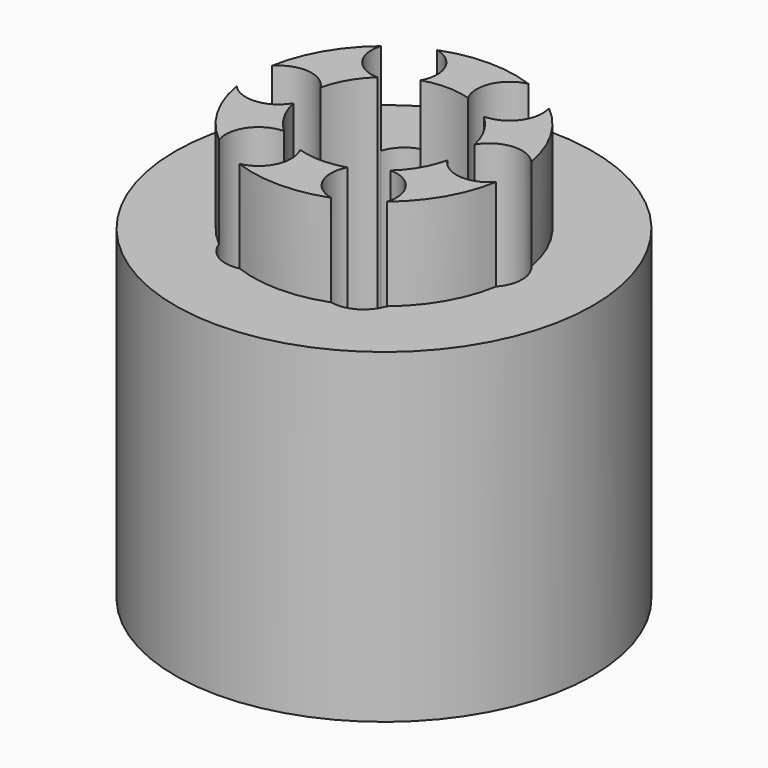
from build123d import *

# Parameters (mm, degrees)
F1_DEPTH = 3.175
F0_R     = 1.5875
F2_DEPTH = 2.475


# Not quite as in the source:
# - a length typed as a fraction of an inch, garbled in the dataset ("3 / 203.2 mm" for 3/8 in), is restored


with BuildPart() as f1:
    # F0 (on Top) → F1 (new body)
    with BuildSketch(Plane.XY):
        with BuildLine():
            ThreePointArc((-0.5859375, 0.1291404123), (-0.5196152423, 0.3), (-0.4048076277, 0.4428665539))
            ThreePointArc((-0.4048076277, 0.4428665539), (-0.6037234698, 0.5479177769), (-0.6376941264, 0.7702896865))
            ThreePointArc((-0.6376941264, 0.7702896865), (-0.8660254038, 0.5), (-0.9859375, 0.16711447))
            ThreePointArc((-0.9859375, 0.16711447), (-0.7763724489, 0.2488809732), (-0.5859375, 0.1291404123))
        make_face()
    extrude(amount=F1_DEPTH)



with BuildPart() as f1b:
    # F0 (on Top) → F1, piece 2 (new body)
    with BuildSketch(Plane.XY):
        with BuildLine():
            ThreePointArc((-0.1811298723, 0.5720069662), (0, 0.6), (0.1811298723, 0.5720069662))
            ThreePointArc((0.1811298723, 0.5720069662), (0.1726489791, 0.7967987502), (0.3482433736, 0.9374041566))
            ThreePointArc((0.3482433736, 0.9374041566), (0, 1), (-0.3482433736, 0.9374041566))
            ThreePointArc((-0.3482433736, 0.9374041566), (-0.2057847115, 0.8502383071), (-0.15, 0.692820323))
            ThreePointArc((-0.15, 0.692820323), (-0.157907526, 0.6304405664), (-0.1811298723, 0.5720069662))
        make_face()
    extrude(amount=F1_DEPTH)


with BuildPart() as f1c:
    # F0 (on Top) → F1, piece 3 (new body)
    with BuildSketch(Plane.XY):
        with BuildLine():
            ThreePointArc((0.4048076277, 0.4428665539), (0.5196152423, 0.3), (0.5859375, 0.1291404123))
            ThreePointArc((0.5859375, 0.1291404123), (0.7763724489, 0.2488809732), (0.9859375, 0.16711447))
            ThreePointArc((0.9859375, 0.16711447), (0.8660254038, 0.5), (0.6376941264, 0.7702896865))
            ThreePointArc((0.6376941264, 0.7702896865), (0.6469043657, 0.732040652), (0.65, 0.692820323))
            ThreePointArc((0.65, 0.692820323), (0.5784683542, 0.5177516321), (0.4048076277, 0.4428665539))
        make_face()
    extrude(amount=F1_DEPTH)


with BuildPart() as f1d:
    # F0 (on Top) → F1, piece 4 (new body)
    with BuildSketch(Plane.XY):
        with BuildLine():
            ThreePointArc((0.9859375, -0.16711447), (0.7763724489, -0.2488809732), (0.5859375, -0.1291404123))
            ThreePointArc((0.5859375, -0.1291404123), (0.5196152423, -0.3), (0.4048076277, -0.4428665539))
            ThreePointArc((0.4048076277, -0.4428665539), (0.5784683542, -0.5177516321), (0.65, -0.692820323))
            ThreePointArc((0.65, -0.692820323), (0.6469043657, -0.732040652), (0.6376941264, -0.7702896865))
            ThreePointArc((0.6376941264, -0.7702896865), (0.8660254038, -0.5), (0.9859375, -0.16711447))
        make_face()
    extrude(amount=F1_DEPTH)


with BuildPart() as f1e:
    # F0 (on Top) → F1, piece 5 (new body)
    with BuildSketch(Plane.XY):
        with BuildLine():
            ThreePointArc((0.3482433736, -0.9374041566), (0.1726489791, -0.7967987502), (0.1811298723, -0.5720069662))
            ThreePointArc((0.1811298723, -0.5720069662), (0, -0.6), (-0.1811298723, -0.5720069662))
            ThreePointArc((-0.1811298723, -0.5720069662), (-0.157907526, -0.6304405664), (-0.15, -0.692820323))
            ThreePointArc((-0.15, -0.692820323), (-0.2057847115, -0.8502383071), (-0.3482433736, -0.9374041566))
            ThreePointArc((-0.3482433736, -0.9374041566), (0, -1), (0.3482433736, -0.9374041566))
        make_face()
    extrude(amount=F1_DEPTH)


with BuildPart() as f1f:
    # F0 (on Top) → F1, piece 6 (new body)
    with BuildSketch(Plane.XY):
        with BuildLine():
            ThreePointArc((-0.6376941264, -0.7702896865), (-0.6037234698, -0.5479177769), (-0.4048076277, -0.4428665539))
            ThreePointArc((-0.4048076277, -0.4428665539), (-0.5196152423, -0.3), (-0.5859375, -0.1291404123))
            ThreePointArc((-0.5859375, -0.1291404123), (-0.7763724489, -0.2488809732), (-0.9859375, -0.16711447))
            ThreePointArc((-0.9859375, -0.16711447), (-0.8660254038, -0.5), (-0.6376941264, -0.7702896865))
        make_face()
    extrude(amount=F1_DEPTH)


with BuildPart() as f1_1:
    add(f1.part)

    add(f1b.part)  # F2 merges F1b

    add(f1c.part)  # F2 merges F1c

    add(f1d.part)  # F2 merges F1d

    add(f1e.part)  # F2 merges F1e

    add(f1f.part)  # F2 merges F1f
    # F0 (on Top) → F2 (join)
    with BuildSketch(Plane.XY):
        Circle(F0_R)
        with BuildLine():
            ThreePointArc((0.6376941264, 0.7702896865), (0.8660254038, 0.5), (0.9859375, 0.16711447))
            ThreePointArc((0.9859375, 0.16711447), (1.0334356175, 0.0894863816), (1.05, 0))
            ThreePointArc((1.05, 0), (1.0334356175, -0.0894863816), (0.9859375, -0.16711447))
            ThreePointArc((0.9859375, -0.16711447), (0.8660254038, -0.5), (0.6376941264, -0.7702896865))
            ThreePointArc((0.6376941264, -0.7702896865), (0.525, -0.909326674), (0.3482433736, -0.9374041566))
            ThreePointArc((0.3482433736, -0.9374041566), (0, -1), (-0.3482433736, -0.9374041566))
            ThreePointArc((-0.3482433736, -0.9374041566), (-0.525, -0.909326674), (-0.6376941264, -0.7702896865))
            ThreePointArc((-0.6376941264, -0.7702896865), (-0.8660254038, -0.5), (-0.9859375, -0.16711447))
            ThreePointArc((-0.9859375, -0.16711447), (-1.05, 0), (-0.9859375, 0.16711447))
            ThreePointArc((-0.9859375, 0.16711447), (-0.8660254038, 0.5), (-0.6376941264, 0.7702896865))
            ThreePointArc((-0.6376941264, 0.7702896865), (-0.525, 0.909326674), (-0.3482433736, 0.9374041566))
            ThreePointArc((-0.3482433736, 0.9374041566), (0, 1), (0.3482433736, 0.9374041566))
            ThreePointArc((0.3482433736, 0.9374041566), (0.525, 0.909326674), (0.6376941264, 0.7702896865))
        make_face(mode=Mode.SUBTRACT)
    extrude(amount=F2_DEPTH)


solid = f1_1.part
